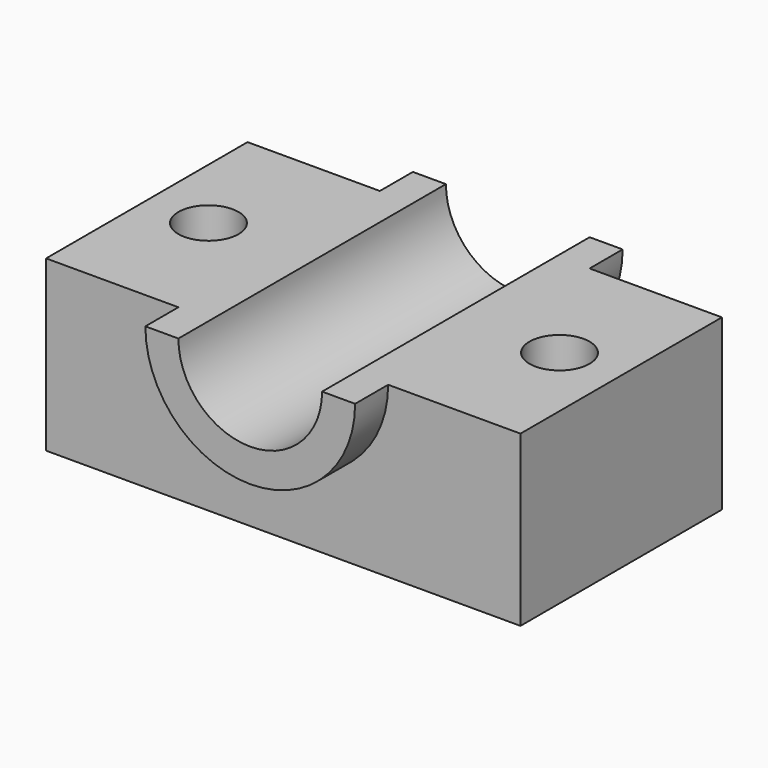
from build123d import *

# Parameters (mm, degrees)
F0_W     = 114.9016693234
F0_H     = 60.9933659434
F0_R     = 7.2773079639
F1_DEPTH = 41
F3_DEPTH = 60.9943659434
F4_DEPTH = 10
F6_DEPTH = 10


with BuildPart() as f1:
    # F0 (on Top) → F1 (new body)
    with BuildSketch(Plane.XY):
        Rectangle(F0_W, F0_H)
        with Locations((-42.510535568, 0)):
            Circle(F0_R, mode=Mode.SUBTRACT)
        with Locations((42.510535568, 0)):
            Circle(F0_R, mode=Mode.SUBTRACT)
    extrude(amount=F1_DEPTH)

    # F2 (on face) → F3 (cut, through all)
    with BuildSketch(Plane.XZ.offset(30.4966829717)):
        with BuildLine():
            ThreePointArc((-17.4030642732, 41), (0, 23.5969357268), (17.4030642732, 41))
            Line((17.4030642732, 41), (-17.4030642732, 41))
        make_face()
    extrude(amount=-F3_DEPTH, mode=Mode.SUBTRACT)

    # F2 (on face) → F4 (join)
    with BuildSketch(Plane.XZ.offset(30.4966829717)):
        with BuildLine():
            Line((25.4030636924, 41), (17.4030642732, 41))
            ThreePointArc((17.4030642732, 41), (0, 23.5969357268), (-17.4030642732, 41))
            Line((-17.4030642732, 41), (-25.4030636924, 41))
            ThreePointArc((-25.4030636924, 41), (0, 15.5969363076), (25.4030636924, 41))
        make_face()
    extrude(amount=F4_DEPTH)

    # F5 (on face) → F6 (join)
    with BuildSketch(Plane(origin=(0, 30.4966829717, 0), x_dir=(-1, 0, 0), z_dir=(0, 1, 0))):
        with BuildLine():
            ThreePointArc((-25.4030636924, 41), (0, 15.5969363076), (25.4030636924, 41))
            Line((25.4030636924, 41), (17.4030642732, 41))
            ThreePointArc((17.4030642732, 41), (0, 23.5969357268), (-17.4030642732, 41))
            Line((-17.4030642732, 41), (-25.4030636924, 41))
        make_face()
    extrude(amount=F6_DEPTH)


solid = f1.part
